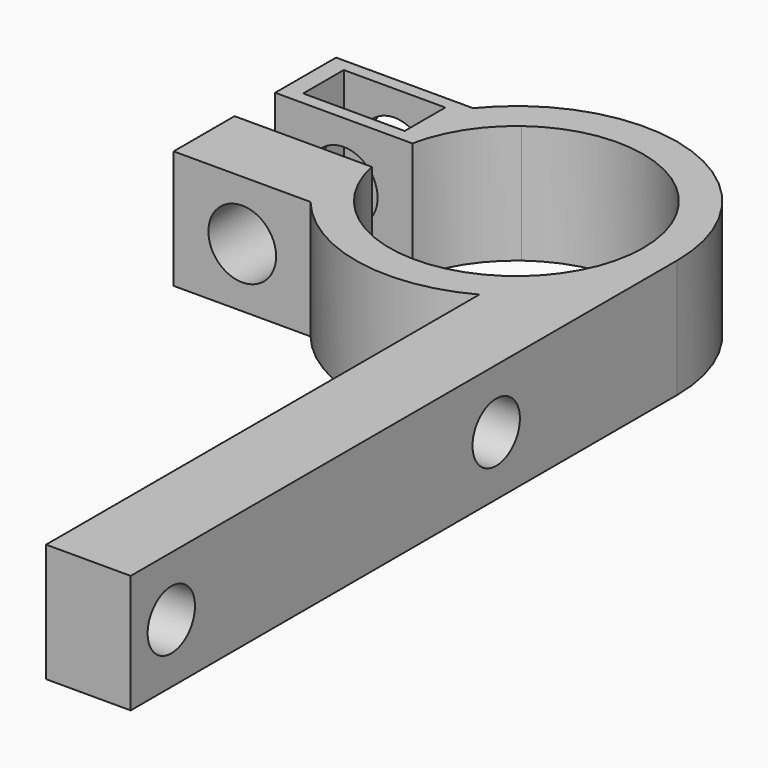
from build123d import *

# Parameters (mm, degrees)
F1_DEPTH      = 7
F2_W          = 6
F2_H          = 3
F3_DEPTH      = 7.001
F4_R          = 1.75
F5_DEPTH      = 5.001
F6_R          = 2
F7_DEPTH      = 4.251
F7_DEPTH_BACK = 45.6176002653


# Not quite as in the source:
# - a feature names something its author has since deleted; it is built from what else it names


with BuildPart() as f1:
    # F0 (on Top) → F1 (new body)
    with BuildSketch(Plane.XY):
        with BuildLine():
            ThreePointArc((-7.3654599313, -6), (-8.6701827743, -3.8830311175), (-9.3808315196, -1.5))
            Line((-9.3808315196, -1.5), (-15.4559988071, -1.5))
            Line((-15.4559988071, -1.5), (-15.4559988071, -6))
            Line((-15.4559988071, -6), (-7.3654599313, -6))
        make_face()
        with BuildLine():
            ThreePointArc((-4.5, 6), (3.3541019662, 6.7082039325), (7.5, 0))
            ThreePointArc((7.5, 0), (0.753817215, -7.4620211475), (-7.3484692283, -1.5))
            Line((-7.3484692283, -1.5), (-9.3808315196, -1.5))
            ThreePointArc((-9.3808315196, -1.5), (-8.6701827743, -3.8830311175), (-7.3654599313, -6))
            ThreePointArc((-7.3654599313, -6), (-1.8582019154, -9.3164953519), (4.5, -8.3666002653))
            ThreePointArc((4.5, -8.3666002653), (8.1547532152, -4.8733971724), (9.5, 0))
            ThreePointArc((9.5, 0), (3.1841899011, 8.9504711984), (-7.3654599313, 6))
            Line((-7.3654599313, 6), (-4.5, 6))
        make_face()
        with BuildLine():
            ThreePointArc((-7.3484692283, 1.5), (-6.3371173071, 4.0113519213), (-4.5, 6))
            Line((-4.5, 6), (-7.3654599313, 6))
            ThreePointArc((-7.3654599313, 6), (-8.6701827743, 3.8830311175), (-9.3808315196, 1.5))
            Line((-9.3808315196, 1.5), (-7.3484692283, 1.5))
        make_face()
        with BuildLine():
            ThreePointArc((-9.3808315196, 1.5), (-8.6701827743, 3.8830311175), (-7.3654599313, 6))
            Line((-7.3654599313, 6), (-15.4559988071, 6))
            Line((-15.4559988071, 6), (-15.4559988071, 1.5))
            Line((-15.4559988071, 1.5), (-9.3808315196, 1.5))
        make_face()
        with BuildLine():
            Line((9.5, -40.3666002653), (9.5, 0))
            ThreePointArc((9.5, 0), (8.1547532152, -4.8733971724), (4.5, -8.3666002653))
            Line((4.5, -8.3666002653), (4.5, -40.3666002653))
            Line((4.5, -40.3666002653), (9.5, -40.3666002653))
        make_face()
    extrude(amount=F1_DEPTH)

    # F2 (on face) → F3 (cut, through all)
    with BuildSketch(Plane.XY.offset(7)):
        with Locations((-11.4022340177, 3.75)):
            Rectangle(F2_W, F2_H)
    extrude(amount=-F3_DEPTH, mode=Mode.SUBTRACT)

    # F4 (on face) → F5 (cut, through all)
    with BuildSketch(Plane(origin=(4.5, 0, 0), x_dir=(0, -1, 0), z_dir=(-1, 0, 0))):
        with Locations((13.3666002653, 3.5)):
            Circle(F4_R)
        with Locations((37.3666002653, 3.5)):
            Circle(F4_R)
    extrude(amount=-F5_DEPTH, mode=Mode.SUBTRACT)

    # F6 (on face) → F7 (cut, two sides)
    with BuildSketch(Plane.XZ.offset(-5.25)) as f7_sk:
        with Locations((-11.4022340177, 3.5)):
            Circle(F6_R)
    extrude(amount=-F7_DEPTH, mode=Mode.SUBTRACT)
    extrude(f7_sk.sketch, amount=F7_DEPTH_BACK, mode=Mode.SUBTRACT)


solid = f1.part
